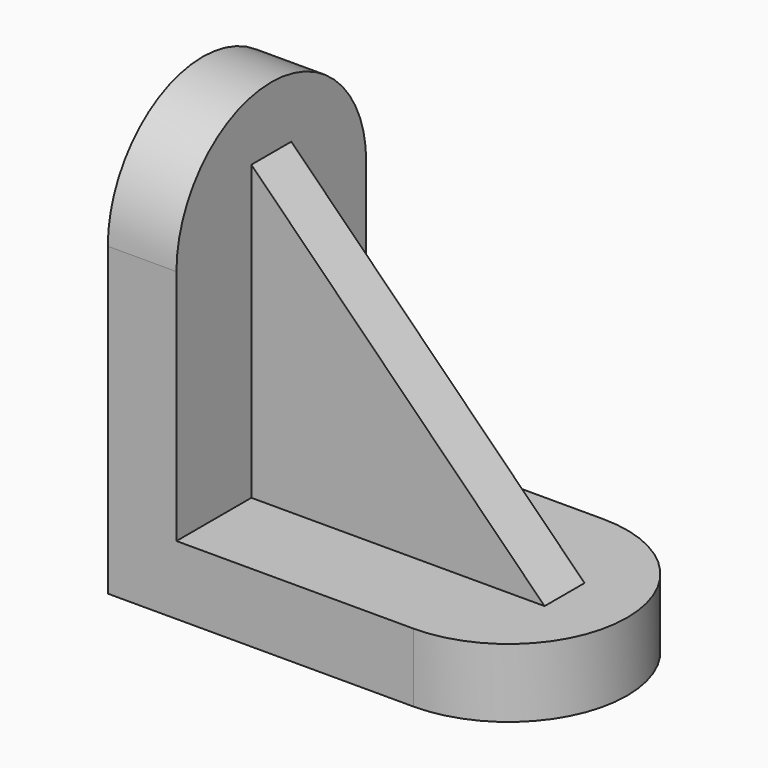
from build123d import *

# Parameters (mm, degrees)
F1_DEPTH    = 38
F3_DEPTH    = 11
F5_DEPTH    = 11
F6_W        = 8
F6_H        = 48.4886
F7_DEPTH    = 48.4886
F8_T4_DEPTH = 265.1682987966


# Not quite as in the source:
# - a fillet or chamfer that OpenCascade refuses, or shapes differently, is made with other operations: its cross-section is extruded or revolved along the edge and cut away or added


with BuildPart() as f1:
    # F0 (on Front) → F1 (new body)
    with BuildSketch(Plane.XZ):
        Polygon((0, 49), (0, 0), (49, 0), (49, 11), (11, 11), (11, 49), align=None)
    extrude(amount=F1_DEPTH)

    # F2 (on face) → F3 (join)
    with BuildSketch(Plane(origin=(0, 0, 0), x_dir=(0, -1, 0), z_dir=(-1, 0, 0))):
        with BuildLine():
            Line((0, 49), (38, 49))
            ThreePointArc((38, 49), (19, 68), (0, 49))
        make_face()
    extrude(amount=-F3_DEPTH)

    # F4 (on face) → F5 (join)
    with BuildSketch(Plane.XY.offset(11)):
        with BuildLine():
            Line((49, 0), (49, -38))
            ThreePointArc((49, -38), (68, -19), (49, 0))
        make_face()
    extrude(amount=-F5_DEPTH)

    # F6 (on face) → F7 (join)
    with BuildSketch(Plane.YZ.offset(11)):
        with Locations((-19, 35.2443)):
            Rectangle(F6_W, F6_H)
    extrude(amount=F7_DEPTH)

    # F8: chamfer of 50 on 1 edges, made by hand


with BuildPart() as f8_tool2:
    # F8_s3 → F8_t4 (new body)
    with BuildSketch(Plane.XZ.offset(-113.5841493983)):
        Polygon((59.4886, 9.4886), (9.4886, 59.4886), (59.4886, 59.4886), align=None)
    extrude(amount=F8_T4_DEPTH)

    split(bisect_by=Plane.XY.offset(11), keep=Keep.TOP)

    split(bisect_by=Plane.YZ.offset(11), keep=Keep.TOP)


with BuildPart() as f1_1:
    add(f1.part)

    # F8_t1: cut F8_tool2
    add(f8_tool2.part, mode=Mode.SUBTRACT)


solid = f1_1.part
